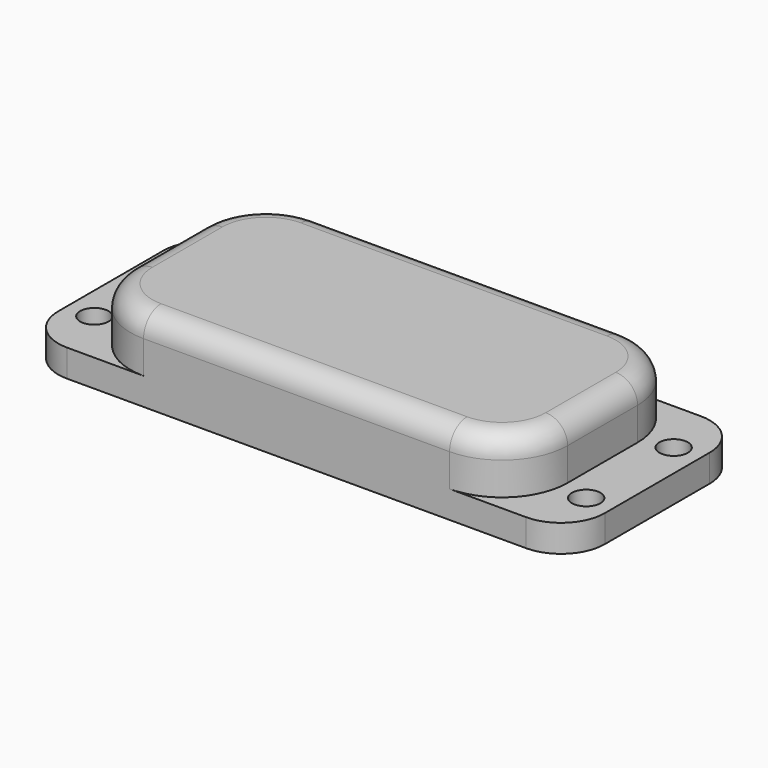
from build123d import *

# Parameters (mm, degrees)
F1_DEPTH     = 25.4
F3_R         = 1.651
F4_DEPTH     = 3.176
F5_R         = 6.35
F6_DEPTH     = 8.89
F7_R         = 5.08
F8_R         = 2.54
F9_T1_DEPTH  = 6.35
F9_T4_ANGLE  = 90
F9_T6_ANGLE  = 90
F9_T8_ANGLE  = 90
F9_T10_ANGLE = 90


# Not quite as in the source:
# - a fillet or chamfer that OpenCascade refuses, or shapes differently, is made with other operations: its cross-section is extruded or revolved along the edge and cut away or added
# - a feature names something its author has since deleted; it is built from what else it names


with BuildPart() as f1:
    # F0 (on Front) → F1 (new body)
    with BuildSketch(Plane.XZ):
        Polygon((-43.9910670578, 3.175), (-43.9910670578, 0), (19.5089329422, 0), (19.5089329422, 3.175), (13.1589329422, 3.175), (13.1589329422, 9.525), (-37.6410670578, 9.525), (-37.6410670578, 3.175), align=None)
    extrude(amount=F1_DEPTH)

    # F3 (on face) → F4 (cut, through all)
    with BuildSketch(Plane.XY.offset(3.175)):
        with Locations((-40.8160670578, -19.05)):
            Circle(F3_R)
        with Locations((-40.8160670578, -6.35)):
            Circle(F3_R)
        with Locations((16.3339329422, -6.35)):
            Circle(F3_R)
        with Locations((16.3339329422, -19.05)):
            Circle(F3_R)
    extrude(amount=-F4_DEPTH, mode=Mode.SUBTRACT)

    # F5 (on face) → F6 (cut)
    with BuildSketch(Plane(origin=(0, 0, 0), x_dir=(1, 0, 0), z_dir=(0, 0, -1))):
        with Locations((-28.7510670578, 12.7)):
            Circle(F5_R)
        with Locations((4.2689329422, 12.7)):
            Circle(F5_R)
        with Locations((-12.2410670578, 12.7)):
            Circle(F5_R)
    extrude(amount=-F6_DEPTH, mode=Mode.SUBTRACT)

    # F7
    f7_edges = [f1.edges().sort_by_distance(p)[0] for p in [
        (19.508933, -25.4, 1.5875),
        (19.508933, 0, 1.5875),
        (-43.991067, -25.4, 1.5875),
        (-43.991067, 0, 1.5875),
    ]]
    fillet(f7_edges, radius=F7_R)

    # F8
    f8_edges = [f1.edges().sort_by_distance(p)[0] for p in [
        (-12.241067, -25.4, 9.525),
        (-37.641067, -12.7, 9.525),
        (-12.241067, 0, 9.525),
        (13.158933, -12.7, 9.525),
    ]]
    fillet(f8_edges, radius=F8_R)

    # F9: fillet of radius 7.62 on 4 edges, made by hand

    # F9_s2 → F9_t1 (cut)
    with BuildSketch(Plane.XY.offset(3.175)):
        with BuildLine():
            ThreePointArc((-37.6410670578, -17.78), (-35.4092207305, -23.1681536726), (-30.0210670578, -25.4))
            Line((-30.0210670578, -25.4), (-37.6410670578, -25.4))
            Line((-37.6410670578, -25.4), (-37.6410670578, -17.78))
        make_face()
        with BuildLine():
            ThreePointArc((13.1589329422, -17.78), (10.9270866148, -23.1681536726), (5.5389329422, -25.4))
            Line((5.5389329422, -25.4), (13.1589329422, -25.4))
            Line((13.1589329422, -25.4), (13.1589329422, -17.78))
        make_face()
        with BuildLine():
            ThreePointArc((-30.0210670578, 0), (-35.4092207305, -2.2318463274), (-37.6410670578, -7.62))
            Line((-37.6410670578, -7.62), (-37.6410670578, 0))
            Line((-37.6410670578, 0), (-30.0210670578, 0))
        make_face()
        with BuildLine():
            ThreePointArc((5.5389329422, 0), (10.9270866148, -2.2318463274), (13.1589329422, -7.62))
            Line((13.1589329422, -7.62), (13.1589329422, 0))
            Line((13.1589329422, 0), (5.5389329422, 0))
        make_face()
    extrude(amount=F9_T1_DEPTH, mode=Mode.SUBTRACT)

    # F9_s3 → F9_t4 (revolve, cut)
    with BuildSketch(Plane.XZ.offset(7.62)):
        with BuildLine():
            ThreePointArc((10.6189329422, 9.525), (12.4149841664, 8.7810512242), (13.1589329422, 6.985))
            Line((13.1589329422, 6.985), (13.1589329422, 9.525))
            Line((13.1589329422, 9.525), (10.6189329422, 9.525))
        make_face()
    revolve(axis=Axis((5.5389329422, -7.62, 9.525), (0, 0, 1)), revolution_arc=F9_T4_ANGLE, mode=Mode.SUBTRACT)

    # F9_s5 → F9_t6 (revolve, cut)
    with BuildSketch(Plane.YZ.offset(-30.0210670578)):
        with BuildLine():
            ThreePointArc((-2.54, 9.525), (-0.7439487758, 8.7810512242), (0, 6.985))
            Line((0, 6.985), (0, 9.525))
            Line((0, 9.525), (-2.54, 9.525))
        make_face()
    revolve(axis=Axis((-30.0210670578, -7.62, 9.525), (0, 0, 1)), revolution_arc=F9_T6_ANGLE, mode=Mode.SUBTRACT)

    # F9_s7 → F9_t8 (revolve, cut)
    with BuildSketch(Plane.YZ.offset(5.5389329422)):
        with BuildLine():
            ThreePointArc((-22.86, 9.525), (-24.6560512242, 8.7810512242), (-25.4, 6.985))
            Line((-25.4, 6.985), (-25.4, 9.525))
            Line((-25.4, 9.525), (-22.86, 9.525))
        make_face()
    revolve(axis=Axis((5.5389329422, -17.78, 9.525), (0, 0, 1)), revolution_arc=F9_T8_ANGLE, mode=Mode.SUBTRACT)

    # F9_s9 → F9_t10 (revolve, cut)
    with BuildSketch(Plane.XZ.offset(17.78)):
        with BuildLine():
            ThreePointArc((-35.1010670578, 9.525), (-36.8971182821, 8.7810512242), (-37.6410670578, 6.985))
            Line((-37.6410670578, 6.985), (-37.6410670578, 9.525))
            Line((-37.6410670578, 9.525), (-35.1010670578, 9.525))
        make_face()
    revolve(axis=Axis((-30.0210670578, -17.78, 9.525), (0, 0, 1)), revolution_arc=F9_T10_ANGLE, mode=Mode.SUBTRACT)


solid = f1.part
